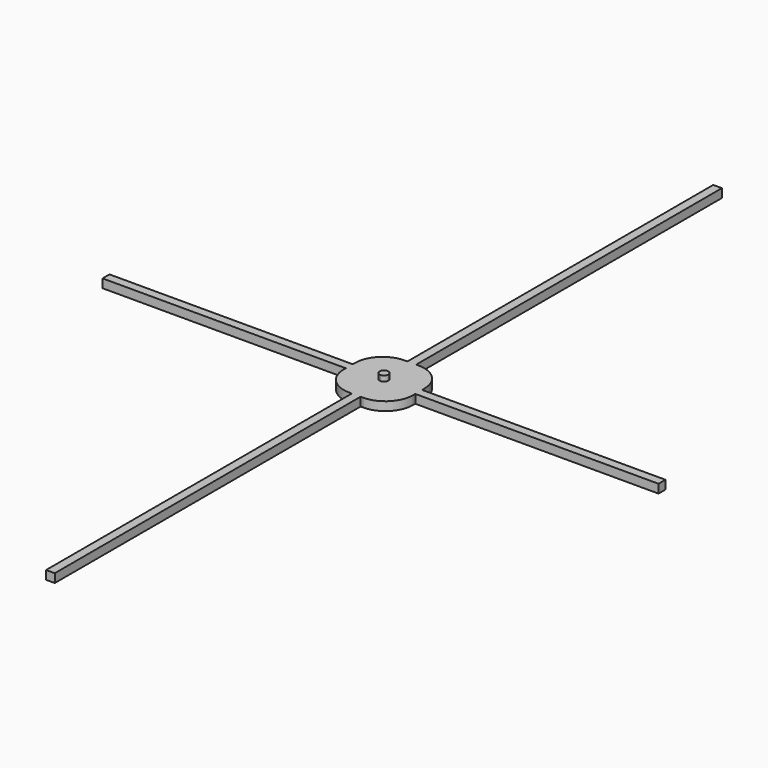
from build123d import *

# Parameters (mm, degrees)
F0_W     = 11.1125013079
F0_H     = 11.1125
F0_W_2   = 3.1749973842
F0_H_2   = 139.7
F0_W_3   = 88.9
F0_H_3   = 3.175
F1_DEPTH = 3.175
F2_DEPTH = 5.1418882795
F3_R     = 10.16


# Not quite as in the source:
# - ends of sketch curves that miss each other by under 0.0002 mm in the source are joined


with BuildPart() as f1:
    # F0 (on Top) → F1 (new body)
    with BuildSketch(Plane.XY):
        with Locations((-7.143749346, 7.14375)):
            Rectangle(F0_W, F0_H)
        with Locations((7.143749346, 7.14375)):
            Rectangle(F0_W, F0_H)
        with Locations((7.143749346, -7.14375)):
            Rectangle(F0_W, F0_H)
        with Locations((-7.143749346, -7.14375)):
            Rectangle(F0_W, F0_H)
        with Locations((0, 82.55)):
            Rectangle(F0_W_2, F0_H_2)
        Polygon((0, 1.5875), (1.5874986921, 1.5875), (1.5874986921, 12.7), (-1.5874986921, 12.7), (-1.5874986921, 1.5875), align=None)
        Polygon((1.5874986921, -1.5875), (12.7, -1.5875), (12.7, 1.5875), (1.5874986921, 1.5875), (1.5874986921, 0), align=None)
        Polygon((-12.7, -1.5875), (-1.5874986921, -1.5875), (-1.5874986921, 0), (-1.5874986921, 1.5875), (-12.7, 1.5875), align=None)
        Polygon((1.5874986921, -12.7), (1.5874986921, -1.5875), (0, -1.5875), (-1.5874986921, -1.5875), (-1.5874986921, -12.7), align=None)
        with Locations((0, -82.55)):
            Rectangle(F0_W_2, F0_H_2)
        with Locations((-57.15, 0)):
            Rectangle(F0_W_3, F0_H_3)
        with Locations((57.15, 0)):
            Rectangle(F0_W_3, F0_H_3)
        with BuildLine():
            Line((-1.5874986921, 1.5875), (-1.5874986921, 0))
            ThreePointArc((-1.5874986921, 0), (-1.1225320151, 1.1225320151), (0, 1.5875))
            Line((0, 1.5875), (-1.5874986921, 1.5875))
        make_face()
        with BuildLine():
            ThreePointArc((-1.5875, 0), (-1.1225320151, -1.1225320151), (0, -1.5875))
            ThreePointArc((0, -1.5875), (1.1225320151, -1.1225320151), (1.5875, 0))
            ThreePointArc((1.5875, 0), (1.1225320151, 1.1225320151), (0, 1.5875))
            ThreePointArc((0, 1.5875), (-1.1225320151, 1.1225320151), (-1.5875, 0))
        make_face()
        with BuildLine():
            ThreePointArc((0, 1.5875), (1.1225320151, 1.1225320151), (1.5875, 0))
            Line((1.5875, 0), (1.5874986921, 1.5875))
            Line((1.5874986921, 1.5875), (0, 1.5875))
        make_face()
        with BuildLine():
            Line((-1.5874986921, -1.5875), (0, -1.5875))
            ThreePointArc((0, -1.5875), (-1.1225320151, -1.1225320151), (-1.5875, 0))
            Line((-1.5875, 0), (-1.5874986921, -1.5875))
        make_face()
        with BuildLine():
            Line((0, -1.5875), (1.5874986921, -1.5875))
            Line((1.5874986921, -1.5875), (1.5874986921, 0))
            ThreePointArc((1.5874986921, 0), (1.1225320151, -1.1225320151), (0, -1.5875))
        make_face()
    extrude(amount=F1_DEPTH)

    # F0 (on Top) → F2 (join)
    with BuildSketch(Plane.XY):
        with BuildLine():
            ThreePointArc((-1.5875, 0), (-1.1225320151, -1.1225320151), (0, -1.5875))
            ThreePointArc((0, -1.5875), (1.1225320151, -1.1225320151), (1.5875, 0))
            ThreePointArc((1.5875, 0), (1.1225320151, 1.1225320151), (0, 1.5875))
            ThreePointArc((0, 1.5875), (-1.1225320151, 1.1225320151), (-1.5875, 0))
        make_face()
    extrude(amount=F2_DEPTH)

    # F3
    f3_edges = [f1.edges().sort_by_distance(p)[0] for p in [
        (12.7, -12.7, 1.5875),
        (-12.7, -12.7, 1.5875),
        (12.7, 12.7, 1.5875),
        (-12.7, 12.7, 1.5875),
    ]]
    fillet(f3_edges, radius=F3_R)


solid = f1.part
